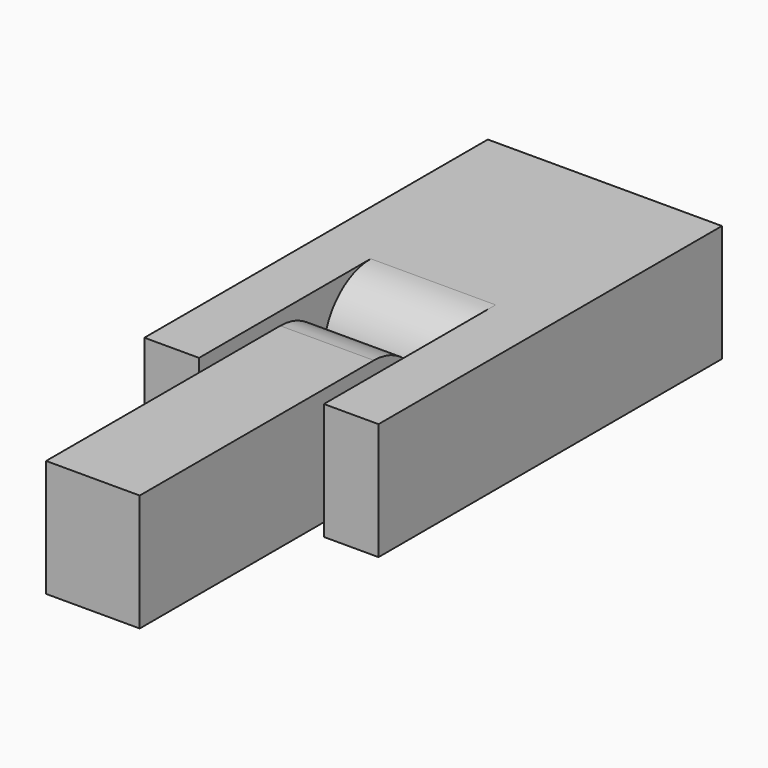
from build123d import *

# Parameters (mm, degrees)
F0_W     = 7
F0_H     = 20
F1_DEPTH = 15
F2_W     = 12
F2_H     = 45
F3_DEPTH = 15
F4_R     = 3.4711759081
F5_DEPTH = 12
F6_R     = 2.4190256098
F7_DEPTH = 30
F8_R     = 7.49999
F8_2_R   = 7.49999


# Not quite as in the source:
# - a fillet or chamfer is up to 0.001 mm smaller than in the source, because OpenCascade refuses the exact size


with BuildPart() as f1:
    # F0 (on Top) → F1 (new body)
    with BuildSketch(Plane.XY):
        Polygon((15, 17.5), (-15, 17.5), (-15, -17.5), (-8, -17.5), (8, -17.5), (15, -17.5), align=None)
        with Locations((-11.5, -27.5)):
            Rectangle(F0_W, F0_H)
        with Locations((11.5, -27.5)):
            Rectangle(F0_W, F0_H)
    extrude(amount=F1_DEPTH)

    # F6 (on face) → F7 (join, through all)
    with BuildSketch(Plane.YZ.offset(15)):
        with Locations((-29.854727909, 6.86943857)):
            Circle(F6_R)
    extrude(amount=-F7_DEPTH)

    # F8 (radius 7.5 in the source; OpenCascade refuses exactly that, so slightly less here)
    f8_edges = [f1.edges().sort_by_distance(p)[0] for p in [
        (0, -17.5, 0),
        (0, -17.5, 15),
    ]]
    fillet(f8_edges, radius=F8_R)


with BuildPart() as f3:
    # F2 (on Top) → F3 (new body)
    with BuildSketch(Plane.XY):
        with Locations((0, -42)):
            Rectangle(F2_W, F2_H)
    extrude(amount=F3_DEPTH)

    # F4 (on face) → F5 (cut, through all)
    with BuildSketch(Plane.YZ.offset(6)):
        with Locations((-29.9282446504, 7.0389099419)):
            Circle(F4_R)
    extrude(amount=-F5_DEPTH, mode=Mode.SUBTRACT)

    # F8#2 (radius 7.5 in the source; OpenCascade refuses exactly that, so slightly less here)
    f8_2_edges = [f3.edges().sort_by_distance(p)[0] for p in [
        (0, -19.5, 0),
        (0, -19.5, 15),
    ]]
    fillet(f8_2_edges, radius=F8_2_R)


solid = Compound([f1.part, f3.part])
